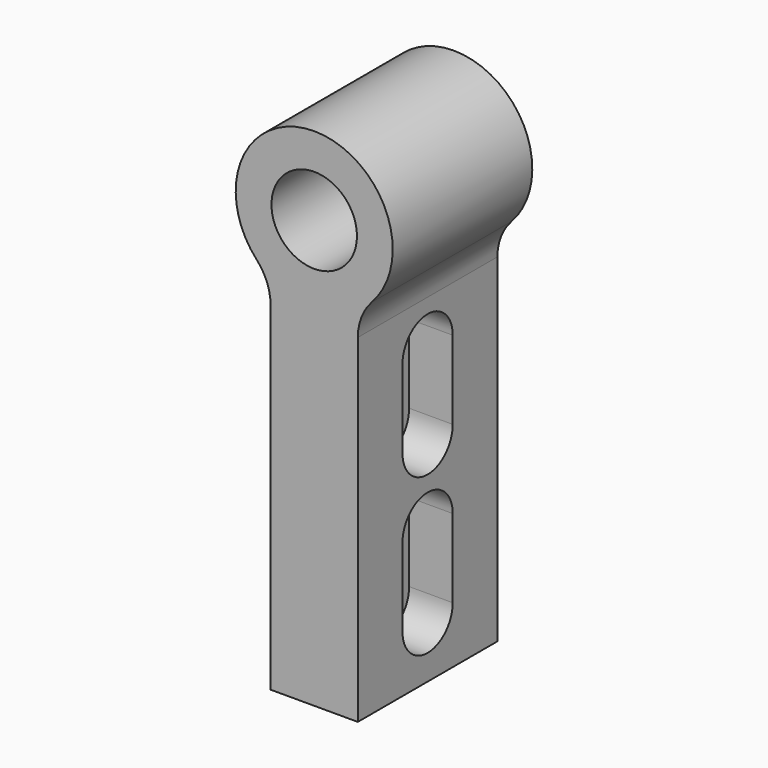
from build123d import *

# Parameters (mm, degrees)
F0_R          = 6.223
F1_DEPTH      = 12.7
F3_R          = 7.62
F2_R          = 2.413
F4_DEPTH      = 17.781
F6_DEPTH      = 17.781
F8_DEPTH      = 6.35
F8_DEPTH_BACK = 5.081


with BuildPart() as f1:
    # F0 (on Front) → F1 (new body, symmetric)
    with BuildSketch(Plane.XZ):
        with BuildLine():
            Line((-6.35, 52.7261902376), (-6.35, 0))
            Line((-6.35, 0), (6.35, 0))
            Line((6.35, 0), (6.35, 52.7261902376))
            ThreePointArc((6.35, 52.7261902376), (0, 73.66), (-6.35, 52.7261902376))
        make_face()
        with Locations((0, 62.23)):
            Circle(F0_R, mode=Mode.SUBTRACT)
    extrude(amount=F1_DEPTH, both=True)

    # F3
    f3_edges = [f1.edges().sort_by_distance(p)[0] for p in [
        (-6.35, 0, 52.72619),
        (6.35, 0, 52.72619),
    ]]
    fillet(f3_edges, radius=F3_R)

    # F2 (on face) → F4 (cut, through all)
    with BuildSketch(Plane.YZ.offset(6.35)):
        with Locations((0, 36.83)):
            Circle(F2_R)
        with Locations((0, 13.97)):
            Circle(F2_R)
    extrude(amount=-F4_DEPTH, mode=Mode.SUBTRACT)

    # F5 (on face) → F6 (cut, through all)
    with BuildSketch(Plane.YZ.offset(6.35)):
        with BuildLine():
            ThreePointArc((2.413, 42.545), (0, 44.958), (-2.413, 42.545))
            Line((-2.413, 42.545), (-2.413, 31.115))
            ThreePointArc((-2.413, 31.115), (0, 28.702), (2.413, 31.115))
            Line((2.413, 31.115), (2.413, 42.545))
        make_face()
        with BuildLine():
            ThreePointArc((2.413, 19.685), (0, 22.098), (-2.413, 19.685))
            Line((-2.413, 19.685), (-2.413, 8.255))
            ThreePointArc((-2.413, 8.255), (0, 5.842), (2.413, 8.255))
            Line((2.413, 8.255), (2.413, 19.685))
        make_face()
    extrude(amount=-F6_DEPTH, mode=Mode.SUBTRACT)

    # F7 (on face) → F8 (cut, two sides)
    with BuildSketch(Plane.YZ.offset(6.35)) as f8_sk:
        with BuildLine():
            Line((4.572, 31.115), (4.572, 42.545))
            ThreePointArc((4.572, 42.545), (0, 47.117), (-4.572, 42.545))
            Line((-4.572, 42.545), (-4.572, 31.115))
            ThreePointArc((-4.572, 31.115), (0, 26.543), (4.572, 31.115))
        make_face()
        with BuildLine():
            Line((4.572, 8.255), (4.572, 19.685))
            ThreePointArc((4.572, 19.685), (0, 24.257), (-4.572, 19.685))
            Line((-4.572, 19.685), (-4.572, 8.255))
            ThreePointArc((-4.572, 8.255), (0, 3.683), (4.572, 8.255))
        make_face()
    extrude(amount=-F8_DEPTH, mode=Mode.SUBTRACT)
    extrude(f8_sk.sketch, amount=F8_DEPTH_BACK, mode=Mode.SUBTRACT)


solid = f1.part
